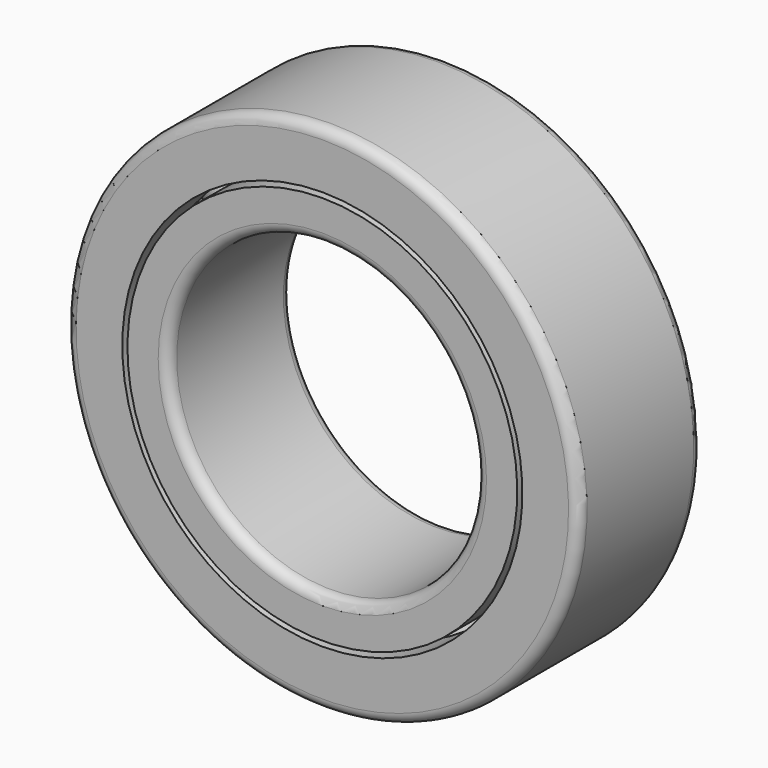
from build123d import *

# Parameters (mm, degrees)
F2_R             = 3
F3_DEPTH         = 3.001
F4_R             = 0.2
F4_2_R           = 0.2
F14_COPIES_COUNT = 3
F14_COPIES_ANGLE = 180


# Not quite as in the source:
# - a feature of the source that left no trace in its solid (it failed there, or was rolled back) is left out
# - a pattern or mirror of a feature is missing from the dataset's text; its kind, count and spacing are read off the source's solid


with BuildPart() as f1:
    # F0 (on Right) → F1 (revolve)
    with BuildSketch(Plane.YZ):
        with BuildLine():
            Line((-1.5, 5), (-1.5, 3.9))
            Line((-1.5, 3.9), (-0.7533923281, 3.9))
            ThreePointArc((-0.7533923281, 3.9), (0, 4.56), (0.7533923281, 3.9))
            Line((0.7533923281, 3.9), (1.5, 3.9))
            Line((1.5, 3.9), (1.5, 5))
            Line((1.5, 5), (-1.5, 5))
        make_face()
    revolve(axis=Axis((0, 0, 0), (0, -1, 0)))

    # F4
    f4_edges = [f1.edges().sort_by_distance(p)[0] for p in [
        (0, 1.5, -5),
        (0, -1.5, -5),
    ]]
    fillet(f4_edges, radius=F4_R)


with BuildPart() as f1b:
    # F0 (on Right) → F1, piece 2 (revolve)
    with BuildSketch(Plane.YZ):
        with BuildLine():
            Line((-1.5, 0), (1.5, 0))
            Line((1.5, 0), (1.5, 3.8))
            Line((1.5, 3.8), (0.76, 3.8))
            ThreePointArc((0.76, 3.8), (0, 3.04), (-0.76, 3.8))
            Line((-0.76, 3.8), (-1.5, 3.8))
            Line((-1.5, 3.8), (-1.5, 0))
        make_face()
    revolve(axis=Axis((0, 0, 0), (0, -1, 0)))

    # F2 (on face) → F3 (cut, through all)
    with BuildSketch(Plane.XZ.offset(1.5)):
        Circle(F2_R)
    extrude(amount=-F3_DEPTH, mode=Mode.SUBTRACT)

    # F4#2
    f4_2_edges = [f1b.edges().sort_by_distance(p)[0] for p in [
        (-3, -1.5, 0),
        (-3, 1.5, 0),
    ]]
    fillet(f4_2_edges, radius=F4_2_R)


with BuildPart() as f6:
    # F5 (on Right) → F6 (revolve)
    with BuildSketch(Plane.YZ):
        with BuildLine():
            Line((-0.75, -3.8), (0.75, -3.8))
            ThreePointArc((0.75, -3.8), (0, -3.05), (-0.75, -3.8))
        make_face()
    revolve(axis=Axis((0, 0, -3.8), (0, -1, 0)))


with BuildPart() as f7_1:
    # F7: instance of F6
    add(f6.part.mirror(Plane.XY))


with BuildPart() as f9:
    # F8 (on Top) → F9 (revolve)
    with BuildSketch(Plane.XY):
        with BuildLine():
            Line((3.8, -0.75), (3.8, 0.75))
            ThreePointArc((3.8, 0.75), (3.05, 0), (3.8, -0.75))
        make_face()
    revolve(axis=Axis((3.8, 0, 0), (0, -1, 0)))


with BuildPart() as f10_1:
    # F10: instance of F9
    add(f9.part.mirror(Plane.YZ))


with BuildPart() as f14:
    # F13 (on face) → F14 (revolve)
    with BuildSketch(Plane(origin=(0, 0, 0), x_dir=(0, 1, 0), z_dir=(0.7071067812, 0, -0.7071067812))):
        with BuildLine():
            Line((-0.75, -3.8), (0.75, -3.8))
            ThreePointArc((0.75, -3.8), (0, -3.05), (-0.75, -3.8))
        make_face()
    revolve(axis=Axis((-2.6870057685, 0, -2.6870057685), (0, 1, 0)))


with BuildPart() as f14_copies_1:
    # F14_copies: instance of F14
    add(f14.part.rotate(Axis((0, 0, 0), (0, 1, 0)), 1 * F14_COPIES_ANGLE / (F14_COPIES_COUNT - 1)))


with BuildPart() as f14_copies_2:
    # F14_copies: instance of F14
    add(f14.part.rotate(Axis((0, 0, 0), (0, 1, 0)), 2 * F14_COPIES_ANGLE / (F14_COPIES_COUNT - 1)))


with BuildPart() as f17:
    # F16 (on face) → F17 (revolve)
    with BuildSketch(Plane(origin=(0, 0, 0), x_dir=(0, 1, 0), z_dir=(0.7071067812, 0, 0.7071067812))):
        with BuildLine():
            Line((-0.75, -3.8), (0.75, -3.8))
            ThreePointArc((0.75, -3.8), (0, -3.05), (-0.75, -3.8))
        make_face()
    revolve(axis=Axis((2.6870057685, 0, -2.6870057685), (0, -1, 0)))


solid = Compound([f1.part, f1b.part, f6.part, f7_1.part, f9.part, f10_1.part, f14.part, f14_copies_1.part, f14_copies_2.part, f17.part])
